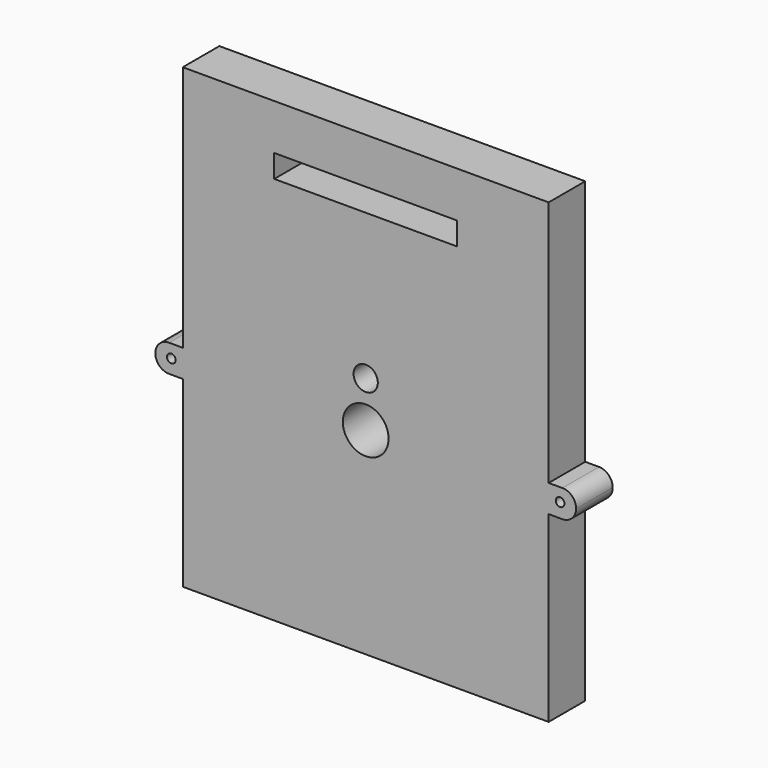
from build123d import *

# Parameters (mm, degrees)
F0_W           = 80
F0_H           = 120
F0_R           = 5
F0_R_2         = 2.65
F1_DEPTH       = 5
F2_W           = 80
F2_H           = 20
F3_DEPTH       = 10
F4_W           = 6
F4_H           = 6
F4_R           = 0.95
F5_DEPTH       = 10
F6_R           = 2.99999
F9_W           = 40
F9_H           = 5
F10_DEPTH      = 12
F10_DEPTH_BACK = 10


# Not quite as in the source:
# - a fillet or chamfer is up to 0.001 mm smaller than in the source, because OpenCascade refuses the exact size


with BuildPart() as f1:
    # F0 (on Front) → F1 (new body, symmetric)
    with BuildSketch(Plane.XZ):
        Rectangle(F0_W, F0_H)
        with Locations((0, 3.126)):
            Circle(F0_R, mode=Mode.SUBTRACT)
        with Locations((0, 13.126)):
            Circle(F0_R_2, mode=Mode.SUBTRACT)
    extrude(amount=F1_DEPTH, both=True)

    # F2 (on face) → F3 (cut)
    with BuildSketch(Plane.XZ.offset(5)):
        with Locations((0, -50)):
            Rectangle(F2_W, F2_H)
    extrude(amount=-F3_DEPTH, mode=Mode.SUBTRACT)

    # F4 (on face) → F5 (join)
    with BuildSketch(Plane.XZ.offset(5)):
        with Locations((43, 3)):
            Rectangle(F4_W, F4_H)
        with Locations((42.5, 3.126)):
            Circle(F4_R, mode=Mode.SUBTRACT)
    extrude(amount=-F5_DEPTH)

    # F6 (radius 3 in the source; OpenCascade refuses exactly that, so slightly less here)
    f6_edges = [f1.edges().sort_by_distance(p)[0] for p in [
        (46, 0, 0),
        (46, 0, 6),
    ]]
    fillet(f6_edges, radius=F6_R)

    # F7: F1 across plane


with BuildPart() as f1_1:
    add(f1.part)
    add(f1.part.mirror(Plane.YZ))

    # F9 (on face) → F10 (cut, two sides)
    with BuildSketch(Plane.XZ.offset(5)) as f10_sk:
        with Locations((0, 47.5)):
            Rectangle(F9_W, F9_H)
    extrude(amount=-F10_DEPTH, mode=Mode.SUBTRACT)
    extrude(f10_sk.sketch, amount=F10_DEPTH_BACK, mode=Mode.SUBTRACT)


solid = f1_1.part
